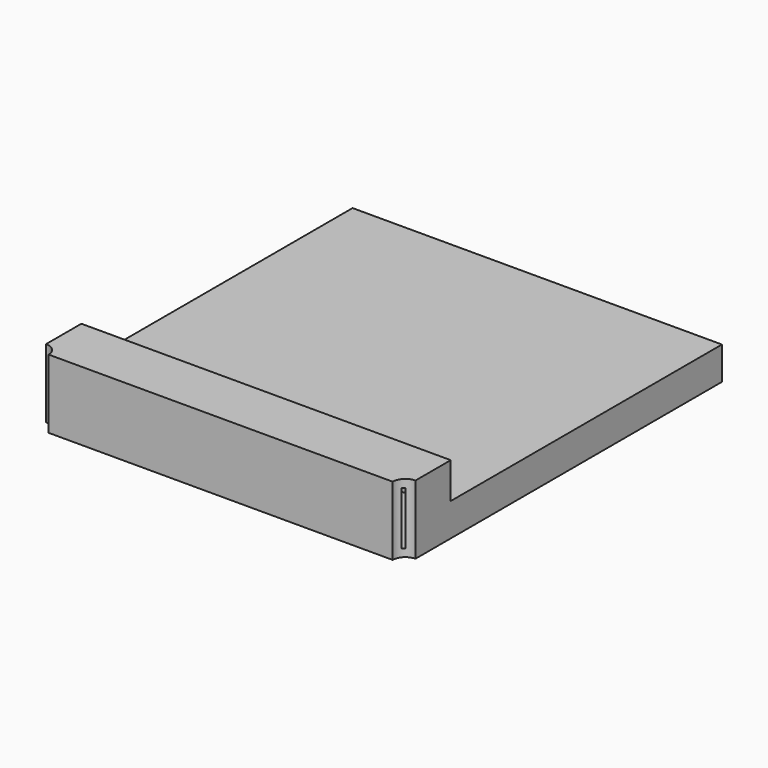
from build123d import *

# Parameters (mm, degrees)
F0_W     = 91.2344232202
F0_H     = 83.7330448863
F1_DEPTH = 8.128
F0_H_2   = 14.015381963
F2_DEPTH = 17.018
F3_T     = -1.9304
F4_D     = 6.2484


# Not quite as in the source:
# - a shell that OpenCascade refuses in one call is made with other operations: the cavity is built on its own and cut out


with BuildPart() as f1:
    # F0 (on Top) → F1 (new body)
    with BuildSketch(Plane.XY):
        with Locations((-8.2024671137, 9.545179052)):
            Rectangle(F0_W, F0_H)
    extrude(amount=F1_DEPTH)

    # F0 (on Top) → F2 (join)
    with BuildSketch(Plane.XY):
        with Locations((-8.2024671137, -39.3290343727)):
            Rectangle(F0_W, F0_H_2)
    extrude(amount=F2_DEPTH)

    # F3: a shell. OpenCascade refuses it in one call, so the cavity is built on its own and cut out:
    # the body offset inwards by the wall thickness, plus a prism from it out through each open face.
    f3_core = offset(f1.part, amount=F3_T, kind=Kind.INTERSECTION, mode=Mode.PRIVATE)
    f3_exits = [f3_core.faces().sort_by_distance(p)[0] for p in [
        (-8.202467, -34.251743, 10.6426),
    ]]
    add(f3_core, mode=Mode.SUBTRACT)
    extrude(f3_exits, amount=-F3_T, mode=Mode.SUBTRACT)

    # F4 (through all)
    with Locations(Plane(origin=(0, 0, 0), x_dir=(1, 0, 0), z_dir=(0, 0, -1))):
        with Locations((37.4147444963, 46.3367253542), (-53.8196787238, 46.3367253542)):
            Hole(F4_D / 2)


solid = f1.part
